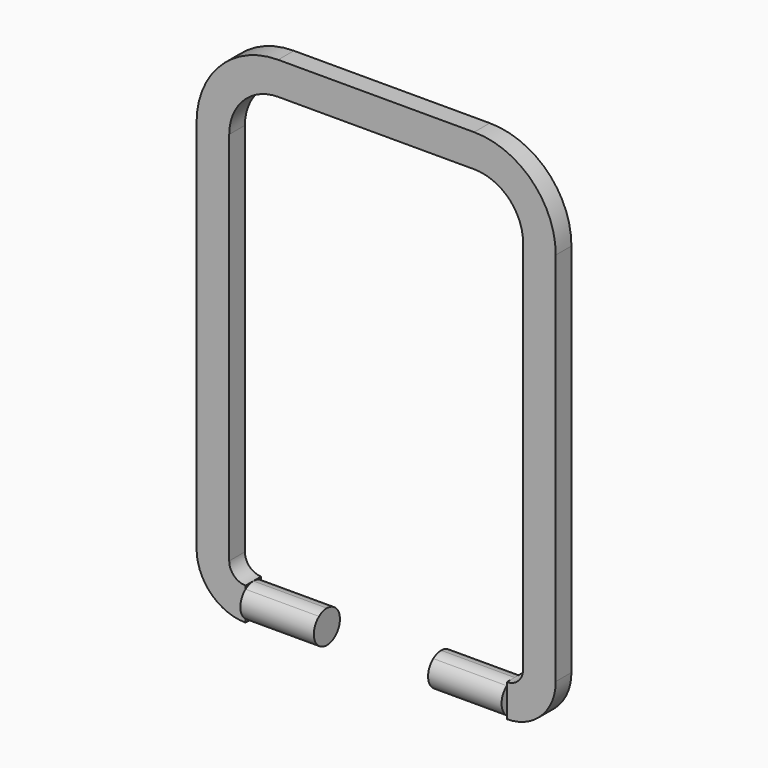
from build123d import *
from build123d import SkipClean  # not in build123d's __all__

# Parameters (mm, degrees)
F1_DEPTH = 1.2
F3_DEPTH = 4.5
F4_DEPTH = 4.5
F6_DEPTH = 4.5
F7_DEPTH = 4.5


with BuildPart() as f1:
    # F0 (on Front) → F1 (new body)
    with BuildSketch(Plane.XZ):
        with BuildLine():
            Line((4.75, 0), (-7.25, 0))
            ThreePointArc((-7.25, 0), (-10.7855339059, -1.4644660941), (-12.25, -5))
            Line((-12.25, -5), (-12.25, -28))
            ThreePointArc((-12.25, -28), (-11.3713203436, -30.1213203436), (-9.25, -31))
            Line((-9.25, -31), (-4.75, -31))
            Line((-4.75, -31), (-4.75, -29))
            Line((-4.75, -29), (-9.25, -29))
            ThreePointArc((-9.25, -29), (-9.9571067812, -28.7071067812), (-10.25, -28))
            Line((-10.25, -28), (-10.25, -5))
            ThreePointArc((-10.25, -5), (-9.3713203436, -2.8786796564), (-7.25, -2))
            Line((-7.25, -2), (4.75, -2))
            ThreePointArc((4.75, -2), (6.8713203436, -2.8786796564), (7.75, -5))
            Line((7.75, -5), (7.75, -28))
            ThreePointArc((7.75, -28), (7.4571067812, -28.7071067812), (6.75, -29))
            Line((6.75, -29), (2.25, -29))
            Line((2.25, -29), (2.25, -31))
            Line((2.25, -31), (6.75, -31))
            ThreePointArc((6.75, -31), (8.8713203436, -30.1213203436), (9.75, -28))
            Line((9.75, -28), (9.75, -5))
            ThreePointArc((9.75, -5), (8.2855339059, -1.4644660941), (4.75, 0))
        make_face()
    extrude(amount=F1_DEPTH)

    # F2 (on face) → F3 (join)
    with BuildSketch(Plane.YZ.offset(-4.75)):
        with BuildLine():
            Line((-1.2, -30.8), (-1.2, -29.2))
            ThreePointArc((-1.2, -29.2), (-1.6, -30), (-1.2, -30.8))
        make_face()
        with BuildLine():
            ThreePointArc((-0.6, -29), (-0.916227766, -29.0513167019), (-1.2, -29.2))
            Line((-1.2, -29.2), (-1.2, -30.8))
            ThreePointArc((-1.2, -30.8), (-0.916227766, -30.9486832981), (-0.6, -31))
            ThreePointArc((-0.6, -31), (-0.283772234, -30.9486832981), (0, -30.8))
            Line((0, -30.8), (0, -29.2))
            ThreePointArc((0, -29.2), (-0.283772234, -29.0513167019), (-0.6, -29))
        make_face()
        with BuildLine():
            ThreePointArc((0.4, -30), (0.294427191, -29.5527864045), (0, -29.2))
            Line((0, -29.2), (0, -30.8))
            ThreePointArc((0, -30.8), (0.294427191, -30.4472135955), (0.4, -30))
        make_face()
    extrude(amount=-F3_DEPTH)

    # F2 (on face) → F4 (cut)
    with BuildSketch(Plane.YZ.offset(-4.75)):
        with BuildLine():
            Line((0, -29), (-0.6, -29))
            ThreePointArc((-0.6, -29), (-0.283772234, -29.0513167019), (0, -29.2))
            Line((0, -29.2), (0, -29))
        make_face()
        with BuildLine():
            Line((-0.6, -29), (-1.2, -29))
            Line((-1.2, -29), (-1.2, -29.2))
            ThreePointArc((-1.2, -29.2), (-0.916227766, -29.0513167019), (-0.6, -29))
        make_face()
        with BuildLine():
            ThreePointArc((0, -30.8), (-0.283772234, -30.9486832981), (-0.6, -31))
            Line((-0.6, -31), (0, -31))
            Line((0, -31), (0, -30.8))
        make_face()
        with BuildLine():
            ThreePointArc((-0.6, -31), (-0.916227766, -30.9486832981), (-1.2, -30.8))
            Line((-1.2, -30.8), (-1.2, -31))
            Line((-1.2, -31), (-0.6, -31))
        make_face()
    with SkipClean():  # cleaning this boolean's faces spoils the solid; the shape is the same uncleaned
        extrude(amount=-F4_DEPTH, mode=Mode.SUBTRACT)

    # F5 (on face) → F6 (join)
    with BuildSketch(Plane(origin=(2.25, 0, 0), x_dir=(0, -1, 0), z_dir=(-1, 0, 0))):
        with BuildLine():
            Line((1.2, -30.8), (1.2, -29.2))
            ThreePointArc((1.2, -29.2), (0.916227766, -29.0513167019), (0.6, -29))
            ThreePointArc((0.6, -29), (0.283772234, -29.0513167019), (0, -29.2))
            Line((0, -29.2), (0, -30.8))
            ThreePointArc((0, -30.8), (0.283772234, -30.9486832981), (0.6, -31))
            ThreePointArc((0.6, -31), (0.916227766, -30.9486832981), (1.2, -30.8))
        make_face()
        with BuildLine():
            Line((0, -30.8), (0, -29.2))
            ThreePointArc((0, -29.2), (-0.4, -30), (0, -30.8))
        make_face()
        with BuildLine():
            ThreePointArc((1.6, -30), (1.494427191, -29.5527864045), (1.2, -29.2))
            Line((1.2, -29.2), (1.2, -30.8))
            ThreePointArc((1.2, -30.8), (1.494427191, -30.4472135955), (1.6, -30))
        make_face()
    extrude(amount=-F6_DEPTH)

    # F5 (on face) → F7 (cut)
    with BuildSketch(Plane(origin=(2.25, 0, 0), x_dir=(0, -1, 0), z_dir=(-1, 0, 0))):
        with BuildLine():
            ThreePointArc((0, -29.2), (0.283772234, -29.0513167019), (0.6, -29))
            Line((0.6, -29), (0, -29))
            Line((0, -29), (0, -29.2))
        make_face()
        with BuildLine():
            Line((1.2, -29.2), (1.2, -29))
            Line((1.2, -29), (0.6, -29))
            ThreePointArc((0.6, -29), (0.916227766, -29.0513167019), (1.2, -29.2))
        make_face()
        with BuildLine():
            Line((0, -31), (0.6, -31))
            ThreePointArc((0.6, -31), (0.283772234, -30.9486832981), (0, -30.8))
            Line((0, -30.8), (0, -31))
        make_face()
        with BuildLine():
            Line((1.2, -31), (1.2, -30.8))
            ThreePointArc((1.2, -30.8), (0.916227766, -30.9486832981), (0.6, -31))
            Line((0.6, -31), (1.2, -31))
        make_face()
    with SkipClean():  # cleaning this boolean's faces spoils the solid; the shape is the same uncleaned
        extrude(amount=-F7_DEPTH, mode=Mode.SUBTRACT)


solid = f1.part
